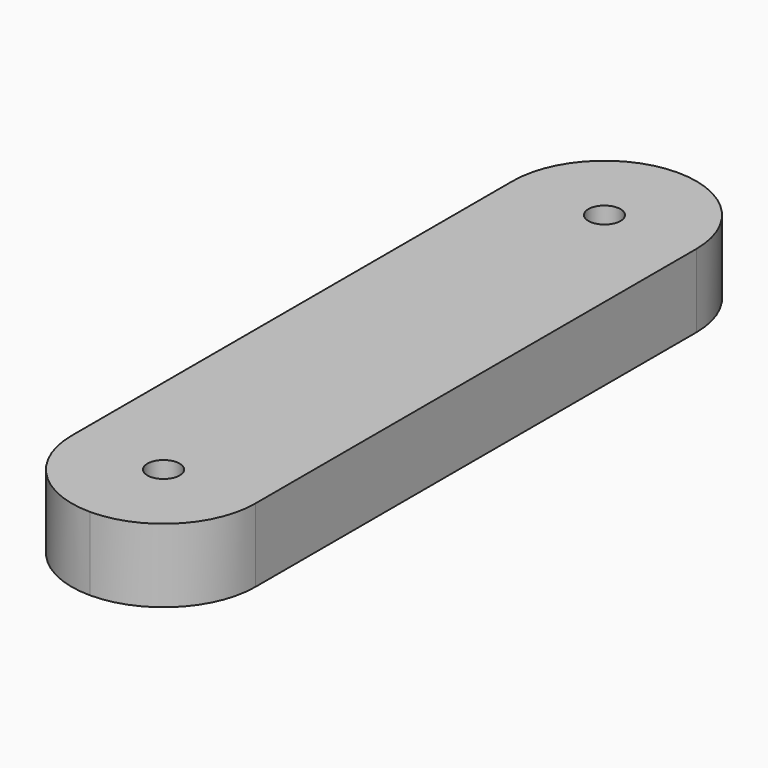
from build123d import *

# Parameters (mm, degrees)
F0_W     = 20
F0_H     = 80
F1_DEPTH = 4
F2_W     = 10
F2_H     = 70
F2_R     = 2.5
F3_DEPTH = 2
F4_R     = 1.75
F5_DEPTH = 8.001
F6_R     = 4.99999
F7_R     = 9.99999


# Not quite as in the source:
# - a fillet or chamfer is up to 0.001 mm smaller than in the source, because OpenCascade refuses the exact size


with BuildPart() as f1:
    # F0 (on Top) → F1 (new body, symmetric)
    with BuildSketch(Plane.XY):
        Rectangle(F0_W, F0_H)
    extrude(amount=F1_DEPTH, both=True)

    # F4 (on face) → F5 (cut, through all)
    with BuildSketch(Plane.XY.offset(4)):
        with Locations((0, 30)):
            Circle(F4_R)
        with Locations((0, -30)):
            Circle(F4_R)
    extrude(amount=-F5_DEPTH, mode=Mode.SUBTRACT)

    # F7 (radius 10 in the source; OpenCascade refuses exactly that, so slightly less here)
    f7_edges = [f1.edges().sort_by_distance(p)[0] for p in [
        (10, 40, 0),
        (-10, 40, 0),
        (-10, -40, 0),
        (10, -40, 0),
    ]]
    fillet(f7_edges, radius=F7_R)


with BuildPart() as f3:
    # F2 (on Top) → F3 (new body, symmetric)
    with BuildSketch(Plane.XY):
        Rectangle(F2_W, F2_H)
        with Locations((0, -30)):
            Circle(F2_R, mode=Mode.SUBTRACT)
        with Locations((0, 30)):
            Circle(F2_R, mode=Mode.SUBTRACT)
    extrude(amount=F3_DEPTH, both=True)

    # F6 (radius 5 in the source; OpenCascade refuses exactly that, so slightly less here)
    f6_edges = [f3.edges().sort_by_distance(p)[0] for p in [
        (5, -35, 0),
        (-5, -35, 0),
        (5, 35, 0),
        (-5, 35, 0),
    ]]
    fillet(f6_edges, radius=F6_R)


with BuildPart() as f1_1:
    add(f1.part)

    # F8: cut F3
    add(f3.part, mode=Mode.SUBTRACT)


solid = Compound([f3.part, f1_1.part])
